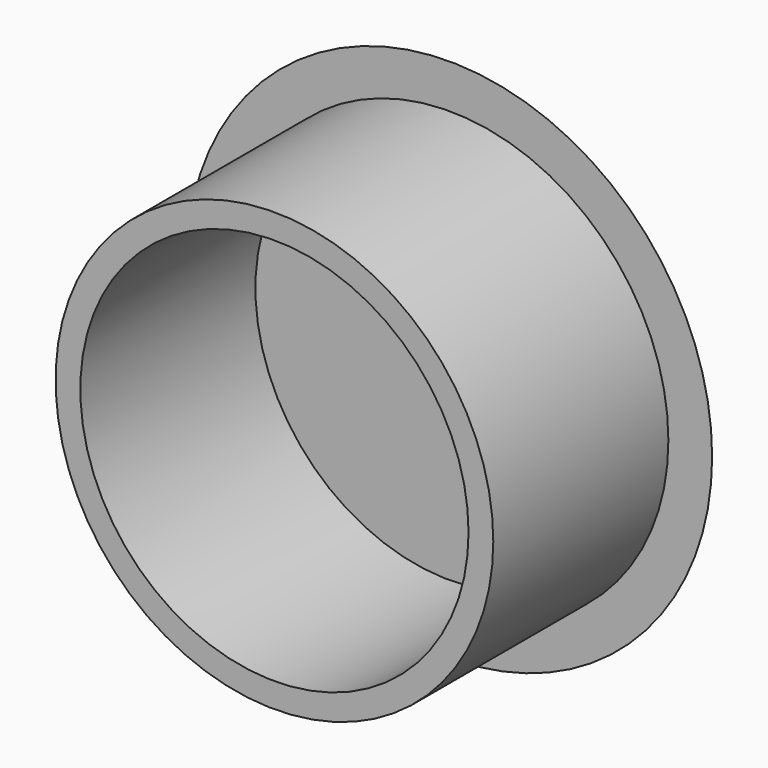
from build123d import *

# Parameters (mm, degrees)
F0_R     = 5
F0_R_2   = 4.4345680592
F1_DEPTH = 5
F2_R     = 6
F3_DEPTH = 1.5


# Not quite as in the source:
# - a fillet or chamfer that OpenCascade refuses, or shapes differently, is made with other operations: its cross-section is extruded or revolved along the edge and cut away or added


with BuildPart() as f1:
    # F0 (on Front) → F1 (new body)
    with BuildSketch(Plane.XZ):
        Circle(F0_R)
        Circle(F0_R_2, mode=Mode.SUBTRACT)
    extrude(amount=F1_DEPTH)

    # F2 (on Front) → F3 (join)
    with BuildSketch(Plane.XZ):
        Circle(F2_R)
    extrude(amount=-F3_DEPTH)

    # F4: fillet of radius 6 on 1 edges, made by hand

    # F4_s1 → F4_t2 (revolve, cut)
    with BuildSketch(Plane.XY):
        with BuildLine():
            ThreePointArc((6, 0), (4.152693377, 1.1124860802), (2.0313730334, 1.5))
            Line((2.0313730334, 1.5), (2.0313730334, 1.62))
            Line((2.0313730334, 1.62), (6, 1.62))
            Line((6, 1.62), (6.12, 1.5))
            ThreePointArc((6.12, 1.5), (6.12, 0.75), (6.0793725393, 0.09))
            Line((6.0793725393, 0.09), (6, 0))
        make_face()
    revolve(axis=Axis((0, 1.5, 0), (0, -1, 0)), mode=Mode.SUBTRACT)


solid = f1.part
